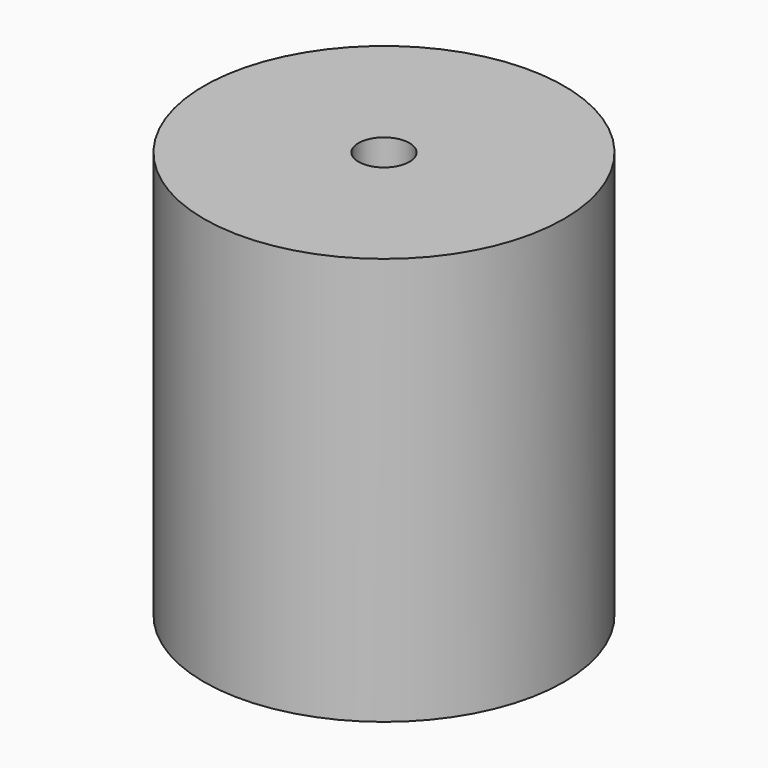
from build123d import *

# Parameters (mm, degrees)
F0_R     = 53
F0_R_2   = 7.5
F2_DEPTH = 120


# Not quite as in the source:
# - the program builds the solid bodies; features that only make, move or delete a surface that nothing else refers to are left out


with BuildPart() as f2:
    # F0 (on Top) → F2 (new body)
    with BuildSketch(Plane.XY):
        Circle(F0_R)
        Circle(F0_R_2, mode=Mode.SUBTRACT)
    extrude(amount=F2_DEPTH)


solid = f2.part
